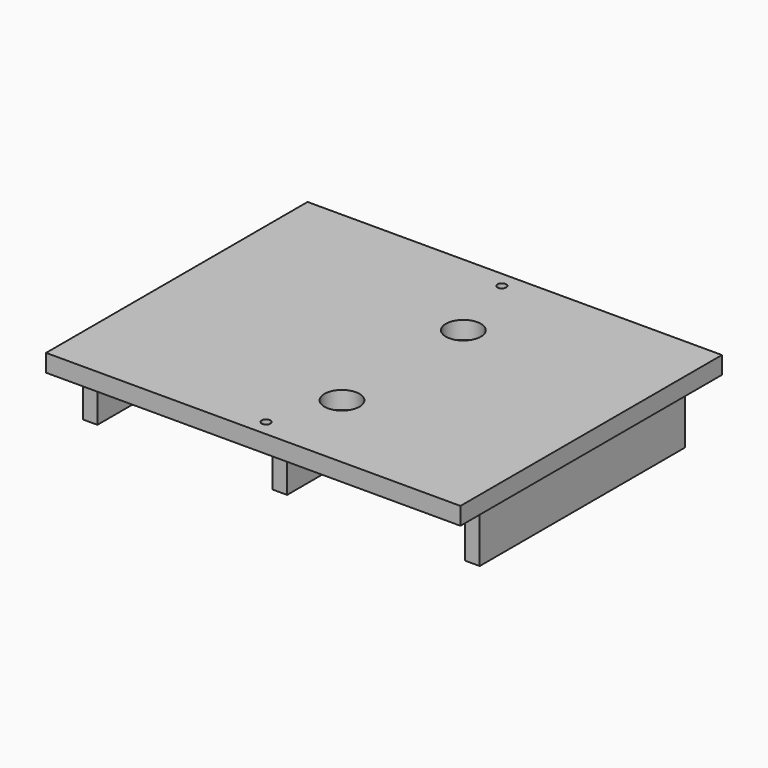
from build123d import *

# Parameters (mm, degrees)
F0_W     = 450.85
F0_H     = 355.6
F1_DEPTH = 19.05
F3_D     = 38.1
F5_D     = 9.525
F6_W     = 15.875
F6_H     = 57.15
F7_DEPTH = 139.7


# Not quite as in the source:
# - a length typed as a fraction of an inch, garbled in the dataset ("3 / 203.2 mm" for 3/8 in), is restored


with BuildPart() as f1:
    # F0 (on Top) → F1 (new body)
    with BuildSketch(Plane.XY):
        Rectangle(F0_W, F0_H)
    extrude(amount=F1_DEPTH)

    # F3 (through all)
    with Locations(Plane.XY.offset(19.05)):
        with Locations((25.4, 76.2), (25.4, -88.9)):
            Hole(F3_D / 2)

    # F5 (through all)
    with Locations(Plane(origin=(0, 0, 0), x_dir=(1, 0, 0), z_dir=(0, 0, -1))):
        with Locations((0, 160.3375), (0, -160.3375)):
            Hole(F5_D / 2)

    # F6 (on Front) → F7 (join, symmetric)
    with BuildSketch(Plane.XZ):
        with Locations((207.9625, -28.575)):
            Rectangle(F6_W, F6_H)
        with Locations((-1.5875, -28.575)):
            Rectangle(F6_W, F6_H)
        with Locations((-207.9625, -28.575)):
            Rectangle(F6_W, F6_H)
    extrude(amount=F7_DEPTH, both=True)


solid = f1.part
